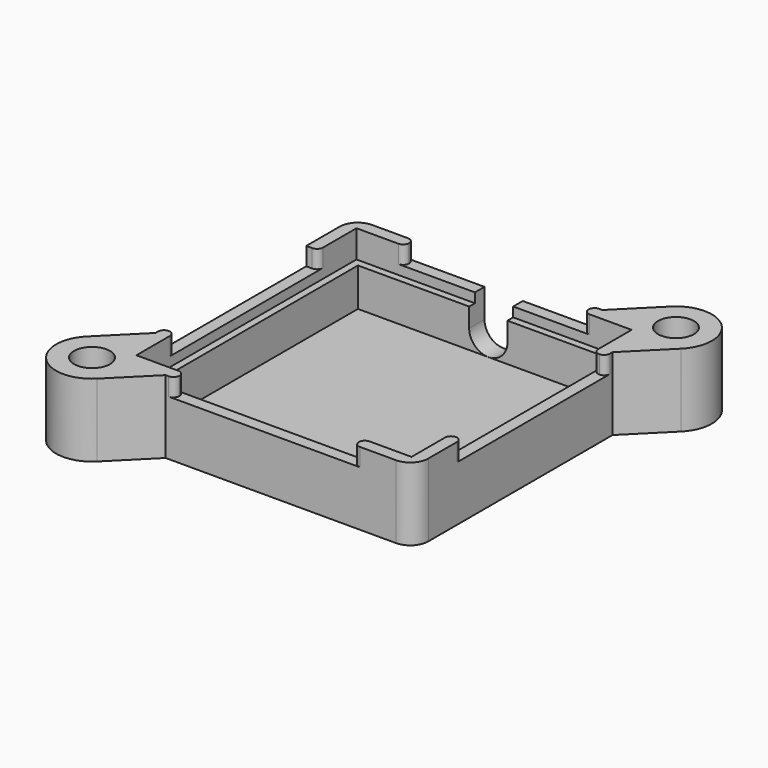
from build123d import *

# Parameters (mm, degrees)
F0_R     = 3
F1_DEPTH = 1.2
F2_R     = 3
F2_W     = 43.6
F2_H     = 43.6
F3_DEPTH = 6.4
F4_R     = 3
F4_W     = 46
F4_H     = 46
F5_DEPTH = 1.6
F6_R     = 3
F7_DEPTH = 3
F9_DEPTH = 3.2
F10_R    = 0.99999
F11_R    = 3


# Not quite as in the source:
# - a fillet or chamfer is up to 0.001 mm smaller than in the source, because OpenCascade refuses the exact size


with BuildPart() as f1:
    # F0 (on Top) → F1 (new body)
    with BuildSketch(Plane.XY):
        with BuildLine():
            Line((22.8786796564, 31.3639610307), (16.5147186258, 25))
            Line((16.5147186258, 25), (-25, 25))
            Line((-25, 25), (-25, -16.5147186258))
            Line((-25, -16.5147186258), (-31.3639610307, -22.8786796564))
            ThreePointArc((-31.3639610307, -22.8786796564), (-31.3639610307, -31.3639610307), (-22.8786796564, -31.3639610307))
            Line((-22.8786796564, -31.3639610307), (-16.5147186258, -25))
            Line((-16.5147186258, -25), (25, -25))
            Line((25, -25), (25, 16.5147186258))
            Line((25, 16.5147186258), (31.3639610307, 22.8786796564))
            ThreePointArc((31.3639610307, 22.8786796564), (31.3639610307, 31.3639610307), (22.8786796564, 31.3639610307))
        make_face()
        with Locations((-27.1213203436, -27.1213203436)):
            Circle(F0_R, mode=Mode.SUBTRACT)
        with Locations((27.1213203436, 27.1213203436)):
            Circle(F0_R, mode=Mode.SUBTRACT)
    extrude(amount=F1_DEPTH)

    # F2 (on face) → F3 (join)
    with BuildSketch(Plane.XY.offset(1.2)):
        with BuildLine():
            Line((-16.5147186258, -25), (25, -25))
            Line((25, -25), (25, 16.5147186258))
            Line((25, 16.5147186258), (31.3639610307, 22.8786796564))
            ThreePointArc((31.3639610307, 22.8786796564), (31.3639610307, 31.3639610307), (22.8786796564, 31.3639610307))
            Line((22.8786796564, 31.3639610307), (16.5147186258, 25))
            Line((16.5147186258, 25), (-25, 25))
            Line((-25, 25), (-25, -16.5147186258))
            Line((-25, -16.5147186258), (-31.3639610307, -22.8786796564))
            ThreePointArc((-31.3639610307, -22.8786796564), (-31.3639610307, -31.3639610307), (-22.8786796564, -31.3639610307))
            Line((-22.8786796564, -31.3639610307), (-16.5147186258, -25))
        make_face()
        with Locations((-27.1213203436, -27.1213203436)):
            Circle(F2_R, mode=Mode.SUBTRACT)
        Rectangle(F2_W, F2_H, mode=Mode.SUBTRACT)
        with Locations((27.1213203436, 27.1213203436)):
            Circle(F2_R, mode=Mode.SUBTRACT)
    extrude(amount=F3_DEPTH)

    # F4 (on face) → F5 (join)
    with BuildSketch(Plane.XY.offset(7.6)):
        with BuildLine():
            Line((-16.5147186258, -25), (25, -25))
            Line((25, -25), (25, 16.5147186258))
            Line((25, 16.5147186258), (31.3639610307, 22.8786796564))
            ThreePointArc((31.3639610307, 22.8786796564), (31.3639610307, 31.3639610307), (22.8786796564, 31.3639610307))
            Line((22.8786796564, 31.3639610307), (16.5147186258, 25))
            Line((16.5147186258, 25), (-25, 25))
            Line((-25, 25), (-25, -16.5147186258))
            Line((-25, -16.5147186258), (-31.3639610307, -22.8786796564))
            ThreePointArc((-31.3639610307, -22.8786796564), (-31.3639610307, -31.3639610307), (-22.8786796564, -31.3639610307))
            Line((-22.8786796564, -31.3639610307), (-16.5147186258, -25))
        make_face()
        with Locations((-27.1213203436, -27.1213203436)):
            Circle(F4_R, mode=Mode.SUBTRACT)
        Rectangle(F4_W, F4_H, mode=Mode.SUBTRACT)
        with Locations((27.1213203436, 27.1213203436)):
            Circle(F4_R, mode=Mode.SUBTRACT)
    extrude(amount=F5_DEPTH)

    # F6 (on face) → F7 (join)
    with BuildSketch(Plane.XY.offset(9.2)):
        Polygon((15, -25), (25, -25), (25, -15), (23, -15), (23, -23), (15, -23), align=None)
        with BuildLine():
            Line((25, 15), (25, 16.5147186258))
            Line((25, 16.5147186258), (31.3639610307, 22.8786796564))
            ThreePointArc((31.3639610307, 22.8786796564), (31.3639610307, 31.3639610307), (22.8786796564, 31.3639610307))
            Line((22.8786796564, 31.3639610307), (16.5147186258, 25))
            Line((16.5147186258, 25), (15, 25))
            Line((15, 25), (15, 23))
            Line((15, 23), (23, 23))
            Line((23, 23), (23, 15))
            Line((23, 15), (25, 15))
        make_face()
        with Locations((27.1213203436, 27.1213203436)):
            Circle(F6_R, mode=Mode.SUBTRACT)
        Polygon((-15, 25), (-25, 25), (-25, 15), (-23, 15), (-23, 23), (-15, 23), align=None)
        with BuildLine():
            Line((-25, -15), (-25, -16.5147186258))
            Line((-25, -16.5147186258), (-31.3639610307, -22.8786796564))
            ThreePointArc((-31.3639610307, -22.8786796564), (-31.3639610307, -31.3639610307), (-22.8786796564, -31.3639610307))
            Line((-22.8786796564, -31.3639610307), (-16.5147186258, -25))
            Line((-16.5147186258, -25), (-15, -25))
            Line((-15, -25), (-15, -23))
            Line((-15, -23), (-23, -23))
            Line((-23, -23), (-23, -15))
            Line((-23, -15), (-25, -15))
        make_face()
        with Locations((-27.1213203436, -27.1213203436)):
            Circle(F6_R, mode=Mode.SUBTRACT)
    extrude(amount=F7_DEPTH)

    # F8 (on face) → F9 (cut, through all)
    with BuildSketch(Plane(origin=(0, 25, 0), x_dir=(-1, 0, 0), z_dir=(0, 1, 0))):
        with BuildLine():
            Line((-3.2, 9.2), (-3.2, 4.4))
            ThreePointArc((-3.2, 4.4), (0, 1.2), (3.2, 4.4))
            Line((3.2, 4.4), (3.2, 9.2))
            Line((3.2, 9.2), (-3.2, 9.2))
        make_face()
    extrude(amount=-F9_DEPTH, mode=Mode.SUBTRACT)

    # F10 (radius 1 in the source; OpenCascade refuses exactly that, so slightly less here)
    f10_edges = [f1.edges().sort_by_distance(p)[0] for p in [
        (25, -15, 10.7),
        (23, -15, 10.7),
        (15, -25, 10.7),
        (15, -23, 10.7),
        (-15, -25, 10.7),
        (-15, -23, 10.7),
        (-23, -15, 10.7),
        (-23, 15, 10.7),
        (-25, -15, 10.7),
        (-15, 23, 10.7),
        (-15, 25, 10.7),
        (15, 23, 10.7),
        (15, 25, 10.7),
        (23, 15, 10.7),
        (25, 15, 10.7),
    ]]
    fillet(f10_edges, radius=F10_R)

    # F11
    f11_edges = [f1.edges().sort_by_distance(p)[0] for p in [
        (-25, 25, 6.1),
        (25, -25, 6.1),
    ]]
    fillet(f11_edges, radius=F11_R)


solid = f1.part
